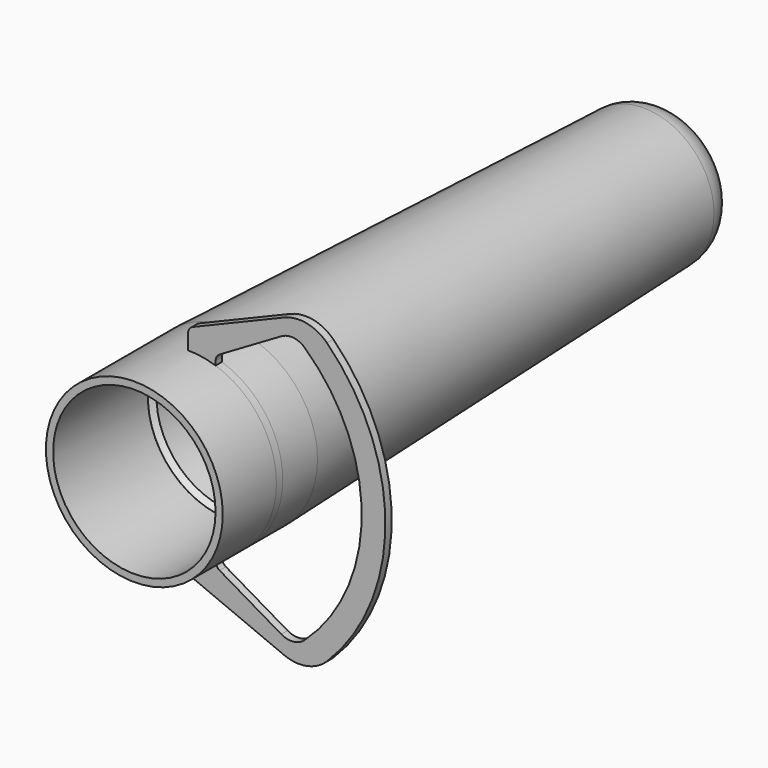
from build123d import *

# Parameters (mm, degrees)
F2_R     = 20.575
F3_DEPTH = 2
F4_R     = 22.4
F4_R_2   = 20.575
F5_DEPTH = 17
F6_DEPTH = 30


# Not quite as in the source:
# - ends of sketch curves that miss each other by under 0.0002 mm in the source are joined


with BuildPart() as f3:
    # F2 (on Front) → F3 (new body)
    with BuildSketch(Plane.XZ):
        with BuildLine():
            Line((-13.8, 76.965483), (-13.8, 73.198817))
            ThreePointArc((-13.8, 73.198817), (-36.2, 50.798817), (-13.8, 28.398817))
            Line((-13.8, 28.398817), (-13.8, 24.63215))
            ThreePointArc((-13.8, 24.63215), (-13.464101, 23.52275), (-12.569231, 22.785996))
            Line((-12.569231, 22.785996), (10.519527, 13.16568))
            ThreePointArc((10.519527, 13.16568), (16.285797, 12.582523), (21.407101, 15.295858))
            ThreePointArc((21.407101, 15.295858), (36.2, 50.798817), (21.407101, 86.301775))
            ThreePointArc((21.407101, 86.301775), (16.285797, 89.01511), (10.519527, 88.431952))
            Line((10.519527, 88.431952), (-12.569231, 78.811637))
            ThreePointArc((-12.569231, 78.811637), (-13.464101, 78.074883), (-13.8, 76.965483))
        make_face()
        with Locations((-13.8, 50.798817)):
            Circle(F2_R, mode=Mode.SUBTRACT)
        with BuildLine():
            ThreePointArc((-6.8, 29.520659), (8.6, 50.798817), (-6.8, 72.076975))
            Line((-6.8, 72.076975), (-6.8, 73.151537))
            ThreePointArc((-6.8, 73.151537), (-6.534832, 74.146705), (-5.809641, 74.877986))
            Line((-5.809641, 74.877986), (9.844156, 84.032447))
            ThreePointArc((9.844156, 84.032447), (12.883236, 84.689734), (15.723162, 83.423698))
            ThreePointArc((15.723162, 83.423698), (30.2, 50.798817), (15.723162, 18.173935))
            ThreePointArc((15.723162, 18.173935), (12.883236, 16.907899), (9.844156, 17.565186))
            Line((9.844156, 17.565186), (-5.809641, 26.719647))
            ThreePointArc((-5.809641, 26.719647), (-6.534832, 27.450928), (-6.8, 28.446096))
            Line((-6.8, 28.446096), (-6.8, 29.520659))
        make_face(mode=Mode.SUBTRACT)
    extrude(amount=F3_DEPTH)

    # F4 (on face) → F5 (join)
    with BuildSketch(Plane.XZ.offset(2)):
        with Locations((-13.8, 50.798817)):
            Circle(F4_R)
        with Locations((-13.8, 50.798817)):
            Circle(F4_R_2, mode=Mode.SUBTRACT)
    extrude(amount=F5_DEPTH)

    # F6 (add): a face of the model
    f6_faces = [f3.faces().sort_by_distance(p)[0] for p in [
        (-35.566432, -19, 50.798817),
    ]]
    extrude(f6_faces, amount=-F6_DEPTH)

    # F7 (on plane+point) → F8 (revolve)
    with BuildSketch(Plane.XY.offset(50.798817)):
        with BuildLine():
            Line((6.7625, 11), (8.6, 11))
            Line((8.6, 11), (4.015629, 142.279196))
            ThreePointArc((4.015629, 142.279196), (1.57777, 147.754718), (-3.979497, 150))
            Line((-3.979497, 150), (-13.8, 150))
            Line((-13.8, 150), (-13.8, 148))
            Line((-13.8, 148), (-4.014418, 148))
            ThreePointArc((-4.014418, 148), (-0.541126, 146.596699), (0.982536, 143.174497))
            Line((0.982536, 143.174497), (5.556041, 12.206459))
            Line((5.556041, 12.206459), (6.7625, 11))
        make_face()
    revolve(axis=Axis((-13.8, 149, 50.798817), (0, -1, 0)))


solid = f3.part
